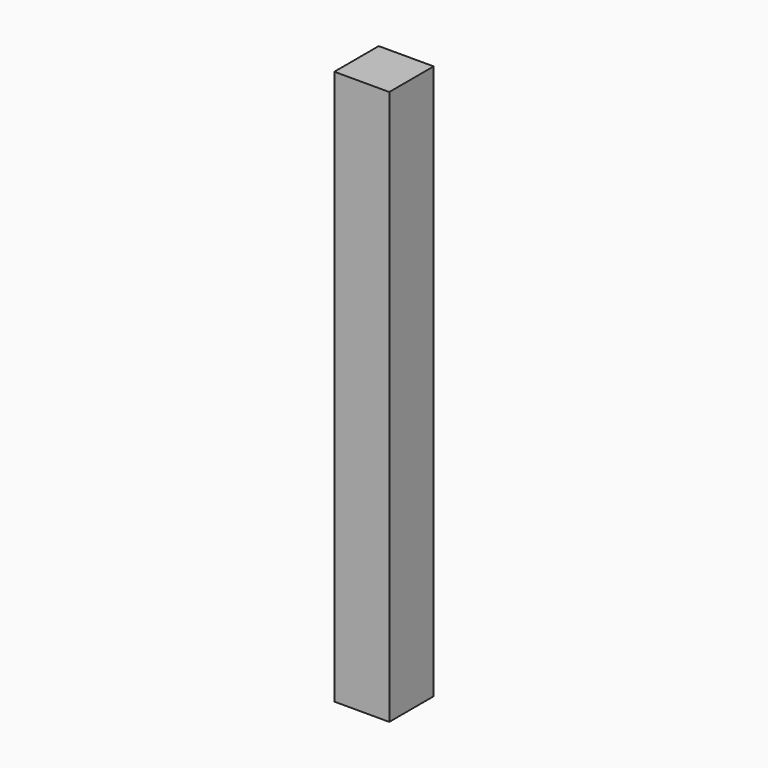
from build123d import *

# Parameters (mm, degrees)
F0_W     = 150.9655937552
F0_H     = 152.5128334761
F1_DEPTH = 1524


# Not quite as in the source:
# - the program builds the solid bodies; features that only make, move or delete a surface that nothing else refers to are left out


with BuildPart() as f1:
    # F0 (on Top) → F1 (new body)
    with BuildSketch(Plane.XY):
        with Locations((0.0875033438, 0.3666356206)):
            Rectangle(F0_W, F0_H)
    extrude(amount=F1_DEPTH)


solid = f1.part
